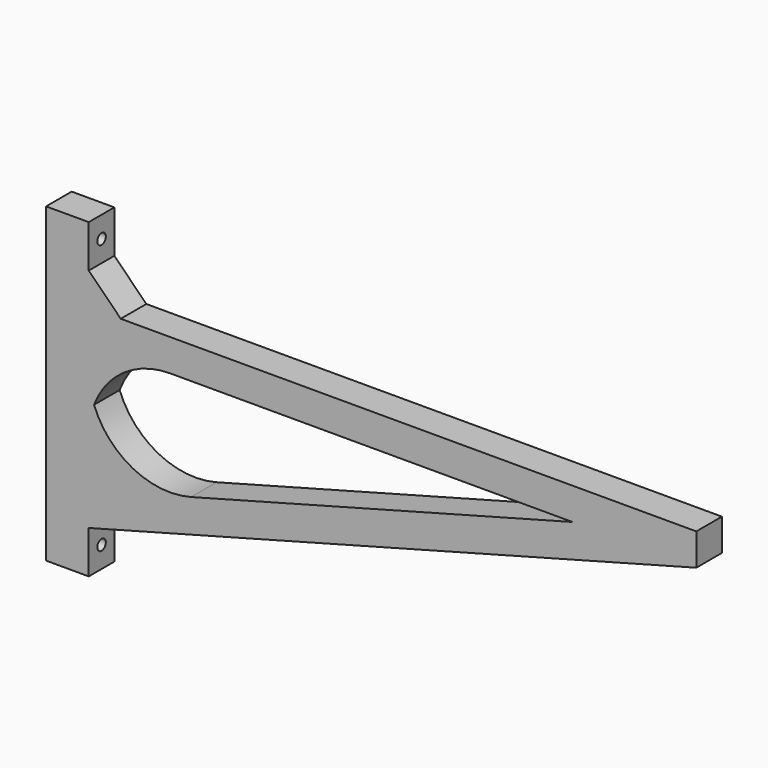
from build123d import *

# Parameters (mm, degrees)
F0_W        = 20
F0_H        = 35
F1_DEPTH    = 15
F2_SIZE     = 15
F3_R        = 2.5
F4_DEPTH    = 20.001
F5_W        = 20
F5_H        = 15
F6_DEPTH    = 20
F7_R        = 2.5
F8_DEPTH    = 20.001
F9_T1_DEPTH = 15


# Not quite as in the source:
# - a fillet or chamfer that OpenCascade refuses, or shapes differently, is made with other operations: its cross-section is extruded or revolved along the edge and cut away or added


with BuildPart() as f1:
    # F0 (on Front) → F1 (new body)
    with BuildSketch(Plane.XZ):
        with Locations((-10, 32.5)):
            Rectangle(F0_W, F0_H)
        Polygon((0, 15), (0, 0), (226.7650184275, 0), (284.8, 0), (284.8, 15), align=None)
        Polygon((284.8, 0), (226.7650184275, 0), (0, -60.6723820371), (0, -76.2), align=None)
        Polygon((0, -60.6723820371), (0, 0), (0, 15), (-20, 15), (-20, -76.2), (0, -76.2), align=None)
    extrude(amount=F1_DEPTH)

    # F2
    f2_edges = [f1.edges().sort_by_distance(p)[0] for p in [
        (0, -7.5, 15),
    ]]
    chamfer(f2_edges, length=F2_SIZE)

    # F3 (on face) → F4 (cut, through all)
    with BuildSketch(Plane.YZ):
        with Locations((-7.5, 40)):
            Circle(F3_R)
    extrude(amount=-F4_DEPTH, mode=Mode.SUBTRACT)

    # F5 (on face) → F6 (join)
    with BuildSketch(Plane(origin=(0, 0, -76.2), x_dir=(1, 0, 0), z_dir=(0, 0, -1))):
        with Locations((-10, 7.5)):
            Rectangle(F5_W, F5_H)
    extrude(amount=F6_DEPTH)

    # F7 (on face) → F8 (cut, through all)
    with BuildSketch(Plane.YZ):
        with Locations((-7.5, -86.2)):
            Circle(F7_R)
    extrude(amount=-F8_DEPTH, mode=Mode.SUBTRACT)

    # F9: fillet of radius 38.1 on 2 edges, made by hand

    # F9_s2 → F9_t1 (join)
    with BuildSketch(Plane.XZ):
        with BuildLine():
            ThreePointArc((0, -11.038341962), (14.9006475381, -41.2608508809), (47.9475089423, -47.8437297148))
            Line((47.9475089423, -47.8437297148), (0, -60.6723820371))
            Line((0, -60.6723820371), (0, -11.038341962))
        make_face()
        with BuildLine():
            ThreePointArc((0, -38.1), (11.1592316368, -11.1592316368), (38.1, 0))
            Line((38.1, 0), (0, 0))
            Line((0, 0), (0, -38.1))
        make_face()
    extrude(amount=F9_T1_DEPTH)


solid = f1.part
